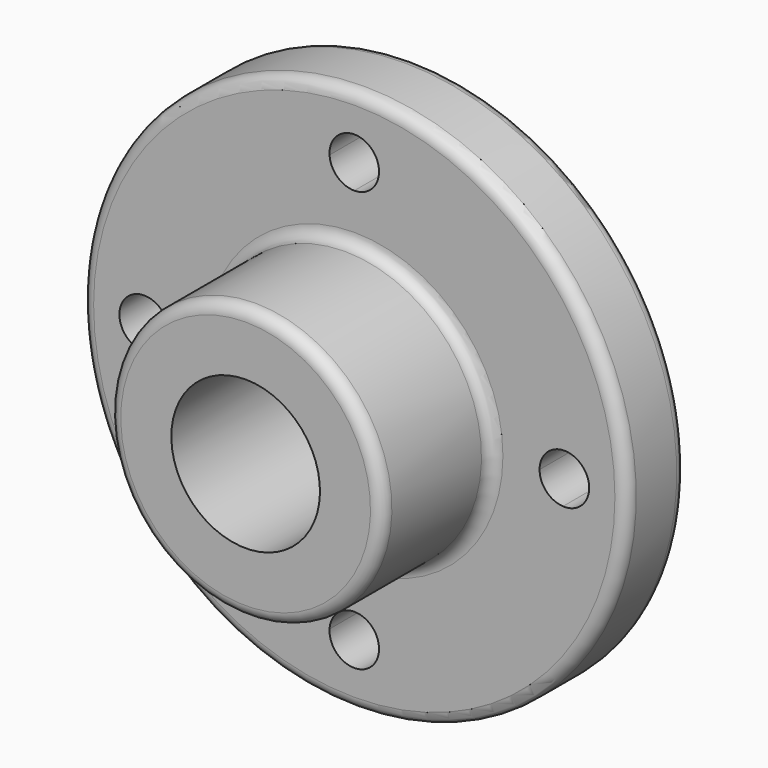
from build123d import *

# Parameters (mm, degrees)
F3_R            = 3.048
F4_DEPTH        = 19.051
F4_COPIES_COUNT = 4


# Not quite as in the source:
# - a pattern or mirror of a feature is missing from the dataset's text; its kind, count and spacing are read off the source's solid


with BuildPart() as f1:
    # F0 (on Right) → F1 (revolve)
    with BuildSketch(Plane.YZ):
        Polygon((-53.848, 19.05), (0, 19.05), (0, 69.85), (-19.05, 69.85), (-19.05, 35.052), (-53.848, 35.052), align=None)
    revolve(axis=Axis((0, -26.924, 0), (0, -1, 0)))

    # F3
    f3_edges = [f1.edges().sort_by_distance(p)[0] for p in [
        (0, -19.05, -69.85),
        (0, 0, -69.85),
        (0, -19.05, -35.052),
        (0, -53.848, -35.052),
    ]]
    fillet(f3_edges, radius=F3_R)

    # F2 (on face) → F4 (cut, through all)
    with BuildSketch(Plane.XZ.offset(19.05)):
        with BuildLine():
            ThreePointArc((-47.498, 0), (-49.2273936601, 4.3557429965), (-53.4735896226, 6.3389523479))
            ThreePointArc((-53.4735896226, 6.3389523479), (-53.848, 0), (-53.4735896226, -6.3389523479))
            ThreePointArc((-53.4735896226, -6.3389523479), (-49.2273936601, -4.3557429965), (-47.498, 0))
        make_face()
        with BuildLine():
            ThreePointArc((-53.4735896226, -6.3389523479), (-53.848, 0), (-53.4735896226, 6.3389523479))
            ThreePointArc((-53.4735896226, 6.3389523479), (-60.198, 0), (-53.4735896226, -6.3389523479))
        make_face()
    f4 = extrude(amount=-F4_DEPTH, mode=Mode.SUBTRACT)

    # F4_copies: F4 ×4 about axis
    f4_copies_axis = Axis((0, 0, 0), (0, 1, 0))
    for i in range(1, F4_COPIES_COUNT):
        add(f4.rotate(f4_copies_axis, i * 360 / F4_COPIES_COUNT), mode=Mode.SUBTRACT)


solid = f1.part
